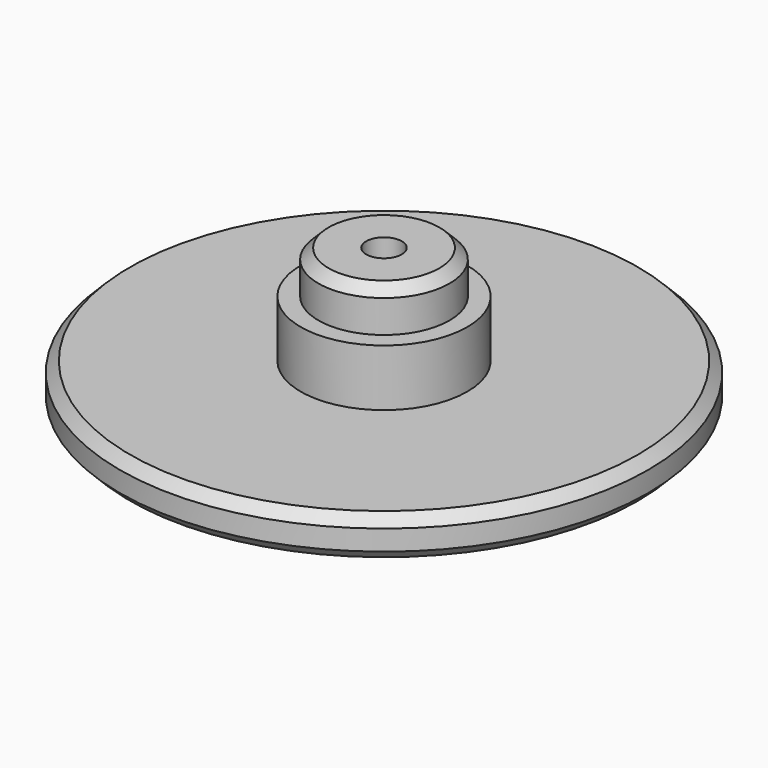
from build123d import *

# Parameters (mm, degrees)
F0_W     = 13
F0_H     = 1
F2_R     = 4.1
F3_DEPTH = 2.8
F4_R     = 3.225
F5_DEPTH = 2.1
F6_R     = 0.875
F7_DEPTH = 5.901
F8_DEPTH = 1
F9_SIZE  = 0.5
F10_SIZE = 2


with BuildPart() as f1:
    # F0 (on Front) → F1 (revolve)
    with BuildSketch(Plane.XZ):
        with Locations((6.5, 0.5)):
            Rectangle(F0_W, F0_H)
    revolve(axis=Axis((0, 0, 1.7087265151), (0, 0, 1)))

    # F2 (on face) → F3 (join)
    with BuildSketch(Plane.XY.offset(1)):
        Circle(F2_R)
    extrude(amount=F3_DEPTH)

    # F4 (on face) → F5 (join)
    with BuildSketch(Plane.XY.offset(3.8)):
        Circle(F4_R)
    extrude(amount=F5_DEPTH)

    # F6 (on face) → F7 (cut, through all)
    with BuildSketch(Plane.XY.offset(5.9)):
        Circle(F6_R)
    extrude(amount=-F7_DEPTH, mode=Mode.SUBTRACT)

    # F8 (add): a face of the model
    f8_faces = [f1.faces().sort_by_distance(p)[0] for p in [
        (-12.6323044738, 0, 0),
    ]]
    extrude(f8_faces, amount=F8_DEPTH)

    # F9
    f9_edges = [f1.edges().sort_by_distance(p)[0] for p in [
        (-13, 0, -1),
        (-13, 0, 1),
        (-3.225, 0, 5.9),
    ]]
    chamfer(f9_edges, length=F9_SIZE)

    # F10
    f10_edges = [f1.edges().sort_by_distance(p)[0] for p in [
        (-0.875, 0, -1),
    ]]
    chamfer(f10_edges, length=F10_SIZE)


solid = f1.part
